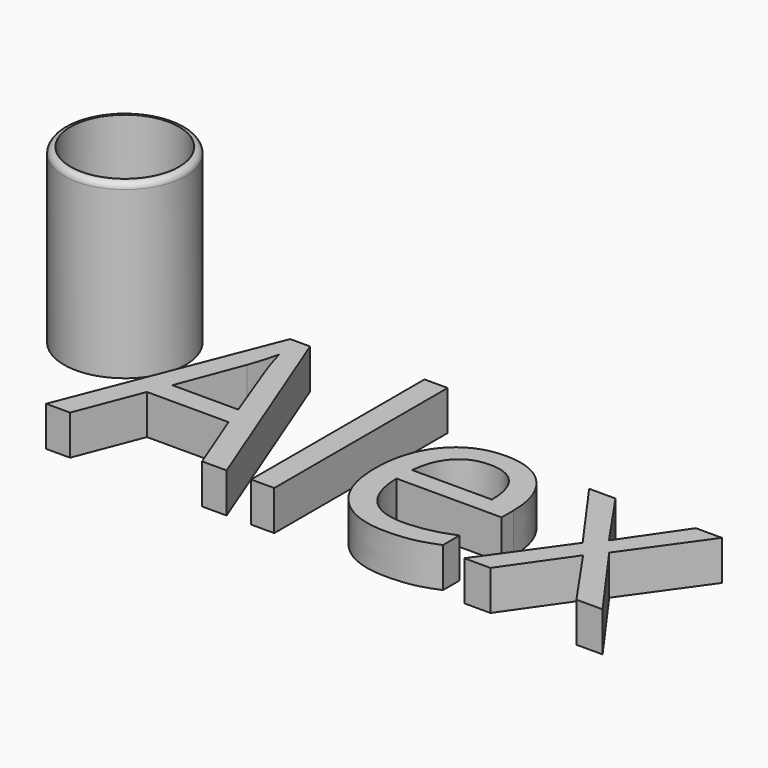
from build123d import *

# Parameters (mm, degrees)
F0_R         = 23.483322854
F1_DEPTH     = 66.5090456605
F2_T         = -2.54
F3_R         = 2.348993721
F4_TEXT_SIZE = 110.1822902759
F5_DEPTH     = 15.3427738696


# Not quite as in the source:
# - Text() gives the source's letters only with a copy of the font that has no kerning and outlines rounded to 1/6400 em; it was checked with that copy


with BuildPart() as f1:
    # F0 (on Top) → F1 (new body)
    with BuildSketch(Plane.XY):
        with Locations((-7.2837024927, 27.6102498174)):
            Circle(F0_R)
    extrude(amount=F1_DEPTH)

    # F2
    f2_openings = [f1.faces().sort_by_distance(p)[0] for p in [
        (-7.283702, 27.61025, 66.509046),
    ]]
    offset(amount=F2_T, openings=f2_openings)

    # F3
    f3_edges = [f1.edges().sort_by_distance(p)[0] for p in [
        (-30.767025, 27.61025, 66.509046),
    ]]
    fillet(f3_edges, radius=F3_R)


with BuildPart() as f5:
    # F4 (on Top) → F5 (new body)
    with BuildSketch(Plane.XY):
        with Locations((17.6181569695, -41.5422320366)):
            Text('Alex', F4_TEXT_SIZE, font='Open Sans', text_align=(TextAlign.LEFT, TextAlign.BOTTOM))
    extrude(amount=F5_DEPTH)


solid = Compound([f1.part, f5.part])
